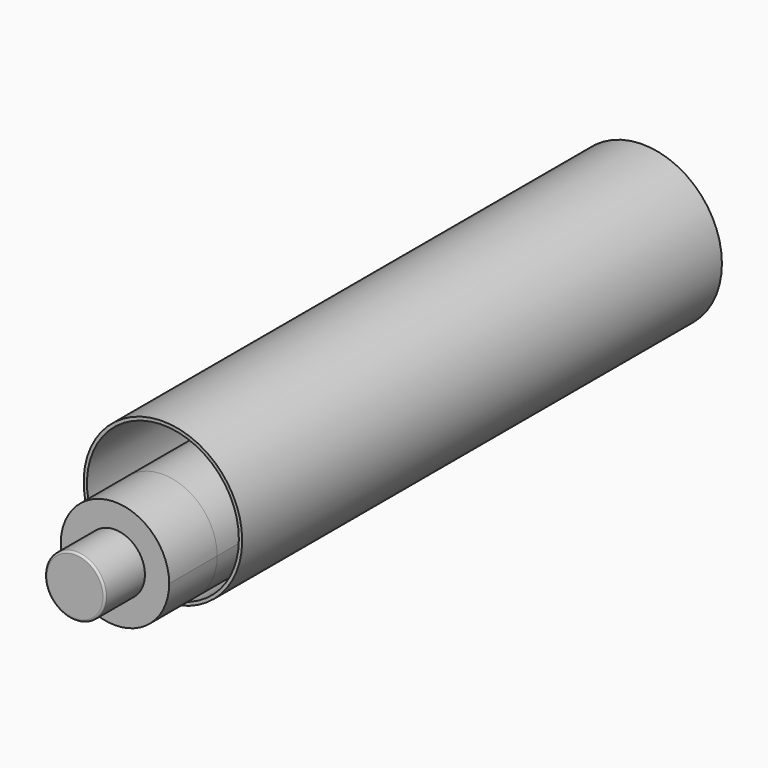
from build123d import *

# Parameters (mm, degrees)
F0_R          = 39.6551273515
F1_DEPTH      = 300
F0_R_2        = 15
F2_DEPTH      = 300
F2_DEPTH_BACK = 30
F3_DEPTH      = 300
F3_DEPTH_BACK = 55
F4_R          = 1


# Not quite as in the source:
# - a feature names something its author has since deleted; it is built from what else it names


with BuildPart() as f1:
    # F0 (on Front) → F1 (new body)
    with BuildSketch(Plane.XZ):
        with Locations((-58.5893206298, 37.1114652178)):
            Circle(F0_R)
        with BuildLine():
            ThreePointArc((-58.5893200762, -0.8885347822), (-85.4593785107, 63.9815227072), (-20.5893206298, 37.1114652178))
            ThreePointArc((-20.5893206298, 37.1114652178), (-31.719262749, 10.2414077285), (-58.5893200762, -0.8885347822))
        make_face(mode=Mode.SUBTRACT)
    extrude(amount=-F1_DEPTH)

    # F0 (on Front) → F2 (join, two sides)
    with BuildSketch(Plane.XZ) as f2_sk:
        with BuildLine():
            ThreePointArc((-31.4543206298, 26.2464652178), (-77.7766633331, 45.4338075296), (-58.5893200762, -0.8885347822))
            ThreePointArc((-58.5893200762, -0.8885347822), (-39.4019779266, 7.0591229061), (-31.4543206298, 26.2464652178))
        make_face()
        with Locations((-58.5893206298, 26.2464652178)):
            Circle(F0_R_2, mode=Mode.SUBTRACT)
    extrude(amount=-F2_DEPTH)
    extrude(f2_sk.sketch, amount=F2_DEPTH_BACK)


with BuildPart() as f3:
    # F0 (on Front) → F3 (new body, two sides)
    with BuildSketch(Plane.XZ) as f3_sk:
        with Locations((-58.5893206298, 26.2464652178)):
            Circle(F0_R_2)
    extrude(amount=-F3_DEPTH)
    extrude(f3_sk.sketch, amount=F3_DEPTH_BACK)

    # F4
    f4_edges = [f3.edges().sort_by_distance(p)[0] for p in [
        (-73.589321, -55, 26.246465),
    ]]
    fillet(f4_edges, radius=F4_R)


solid = Compound([f1.part, f3.part])
